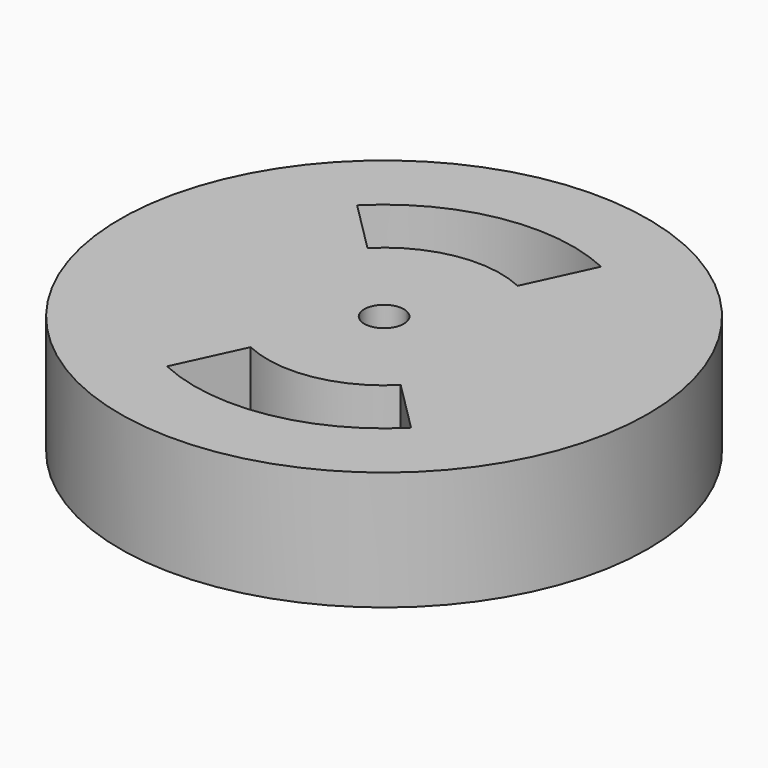
from build123d import *

# Parameters (mm, degrees)
F0_R     = 20
F1_DEPTH = 9


# Not quite as in the source:
# - a feature names something its author has since deleted; it is built from what else it names


with BuildPart() as f1:
    # F0 (on Top) → F1 (new body)
    with BuildSketch(Plane.XY):
        Circle(F0_R)
        with BuildLine():
            Line((-6.0368402564, -13.007011068), (-3.7146515348, -8.0036097652))
            ThreePointArc((-3.7146515348, -8.0036097652), (1.5436452389, -8.6875522833), (6.244462038, -6.2340275228))
            Line((6.244462038, -6.2340275228), (10.1481443029, -10.1311867228))
            ThreePointArc((10.1481443029, -10.1311867228), (2.5086443863, -14.1185155221), (-6.0368402564, -13.007011068))
        make_face(mode=Mode.SUBTRACT)
        with BuildLine():
            Line((6.0368402564, 13.007011068), (3.7146515348, 8.0036097652))
            ThreePointArc((3.7146515348, 8.0036097652), (-1.5436452389, 8.6875522833), (-6.244462038, 6.2340275228))
            Line((-6.244462038, 6.2340275228), (-10.1481443029, 10.1311867228))
            ThreePointArc((-10.1481443029, 10.1311867228), (-2.5086443863, 14.1185155221), (6.0368402564, 13.007011068))
        make_face(mode=Mode.SUBTRACT)
        with BuildLine():
            ThreePointArc((0.6314837286, 1.3605985082), (1.2643626048, 0.8070856234), (1.5, 0))
            ThreePointArc((1.5, 0), (-1.2643626048, -0.8070856234), (0.6314837286, 1.3605985082))
        make_face(mode=Mode.SUBTRACT)
    extrude(amount=F1_DEPTH)


solid = f1.part
